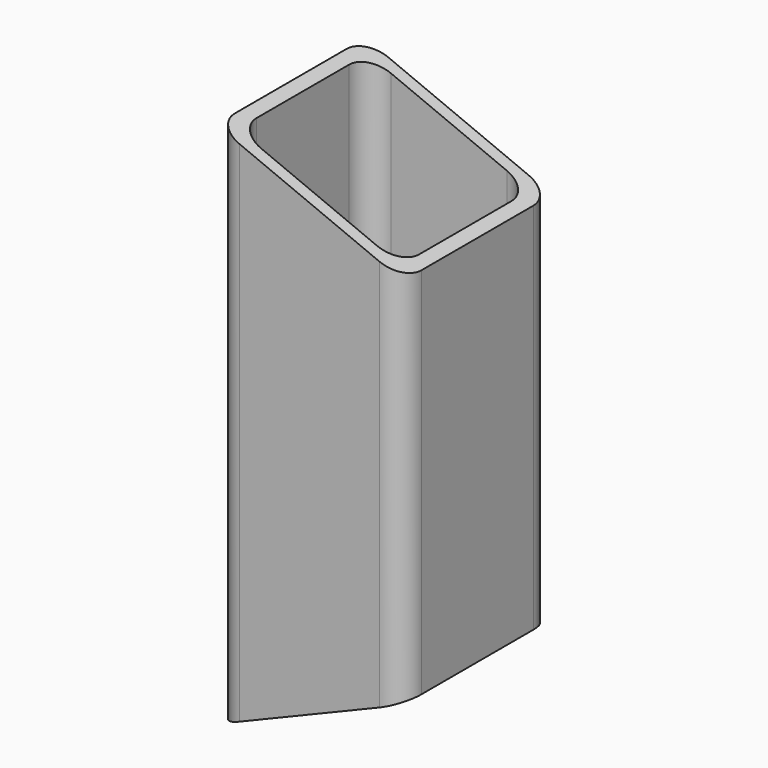
from build123d import *

# Parameters (mm, degrees)
F1_W     = 25.4
F1_H     = 25.4
F2_DEPTH = 71.8312
F4_DEPTH = 25.4
F5_R     = 3.175


# Not quite as in the source:
# - a variable given as a bare number and used for a length is read in inches; the dataset says mm whatever the document's units were
# - a feature names something its author has since deleted; it is built from what else it names


with BuildPart() as f2:
    # F1 (on Top) → F2 (new body)
    with BuildSketch(Plane.XY):
        Rectangle(F1_W, F1_H)
        with BuildLine():
            ThreePointArc((-11.049, 7.874), (-10.1190640303, 10.1190640303), (-7.874, 11.049))
            Line((-7.874, 11.049), (7.874, 11.049))
            ThreePointArc((7.874, 11.049), (10.1190640303, 10.1190640303), (11.049, 7.874))
            Line((11.049, 7.874), (11.049, -7.874))
            ThreePointArc((11.049, -7.874), (10.1190640303, -10.1190640303), (7.874, -11.049))
            Line((7.874, -11.049), (-7.874, -11.049))
            ThreePointArc((-7.874, -11.049), (-10.1190640303, -10.1190640303), (-11.049, -7.874))
            Line((-11.049, -7.874), (-11.049, 7.874))
        make_face(mode=Mode.SUBTRACT)
    extrude(amount=F2_DEPTH)

    # F3 (on face) → F4 (cut)
    with BuildSketch(Plane.XZ.offset(12.7)):
        Polygon((12.7, 10.5210244843), (-12.7, 0), (12.7, 0), align=None)
        Polygon((12.7, 71.8312), (-12.7, 71.8312), (12.7, 61.3101755157), align=None)
    extrude(amount=-F4_DEPTH, mode=Mode.SUBTRACT)

    # F5
    f5_edges = [f2.edges().sort_by_distance(p)[0] for p in [
        (-12.7, 12.7, 35.9156),
        (12.7, 12.7, 35.9156),
        (-12.7, -12.7, 35.9156),
        (12.7, -12.7, 35.9156),
    ]]
    fillet(f5_edges, radius=F5_R)


solid = f2.part
